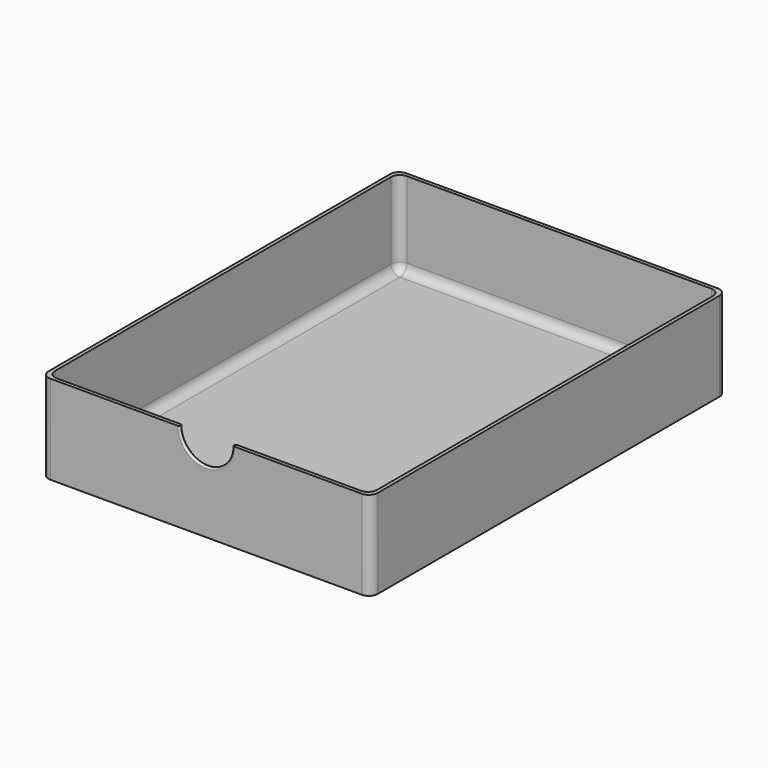
from build123d import *

# Parameters (mm, degrees)
F0_W     = 185
F0_H     = 250
F0_W_2   = 181
F0_H_2   = 246
F1_DEPTH = 50
F2_DEPTH = 2
F3_R     = 5
F4_R     = 5
F5_R     = 15
F6_DEPTH = 25
F7_R     = 0.99999


# Not quite as in the source:
# - a fillet or chamfer is up to 0.001 mm smaller than in the source, because OpenCascade refuses the exact size


with BuildPart() as f1:
    # F0 (on Top) → F1 (new body)
    with BuildSketch(Plane.XY):
        Rectangle(F0_W, F0_H)
        Rectangle(F0_W_2, F0_H_2, mode=Mode.SUBTRACT)
    extrude(amount=F1_DEPTH)

    # F0 (on Top) → F2 (join)
    with BuildSketch(Plane.XY):
        Rectangle(F0_W, F0_H)
        Rectangle(F0_W_2, F0_H_2, mode=Mode.SUBTRACT)
        Rectangle(F0_W_2, F0_H_2)
    extrude(amount=F2_DEPTH)

    # F3
    f3_edges = [f1.edges().sort_by_distance(p)[0] for p in [
        (92.5, 125, 25),
        (-92.5, 125, 25),
        (90.5, 123, 26),
        (-90.5, 123, 26),
        (-90.5, -123, 26),
        (-92.5, -125, 25),
        (92.5, -125, 25),
        (90.5, -123, 26),
    ]]
    fillet(f3_edges, radius=F3_R)

    # F4
    f4_edges = [f1.edges().sort_by_distance(p)[0] for p in [
        (-90.5, 0, 2),
        (-89.035534, -121.535534, 2),
        (-89.035534, 121.535534, 2),
        (0, -123, 2),
        (0, 123, 2),
        (89.035534, -121.535534, 2),
        (89.035534, 121.535534, 2),
        (90.5, 0, 2),
    ]]
    fillet(f4_edges, radius=F4_R)

    # F5 (on face) → F6 (cut)
    with BuildSketch(Plane.XZ.offset(125)):
        with Locations((0, 50)):
            Circle(F5_R)
    extrude(amount=-F6_DEPTH, mode=Mode.SUBTRACT)

    # F7 (radius 1 in the source; OpenCascade refuses exactly that, so slightly less here)
    f7_edges = [f1.edges().sort_by_distance(p)[0] for p in [
        (0, -123, 35),
        (0, -125, 35),
    ]]
    fillet(f7_edges, radius=F7_R)


solid = f1.part
